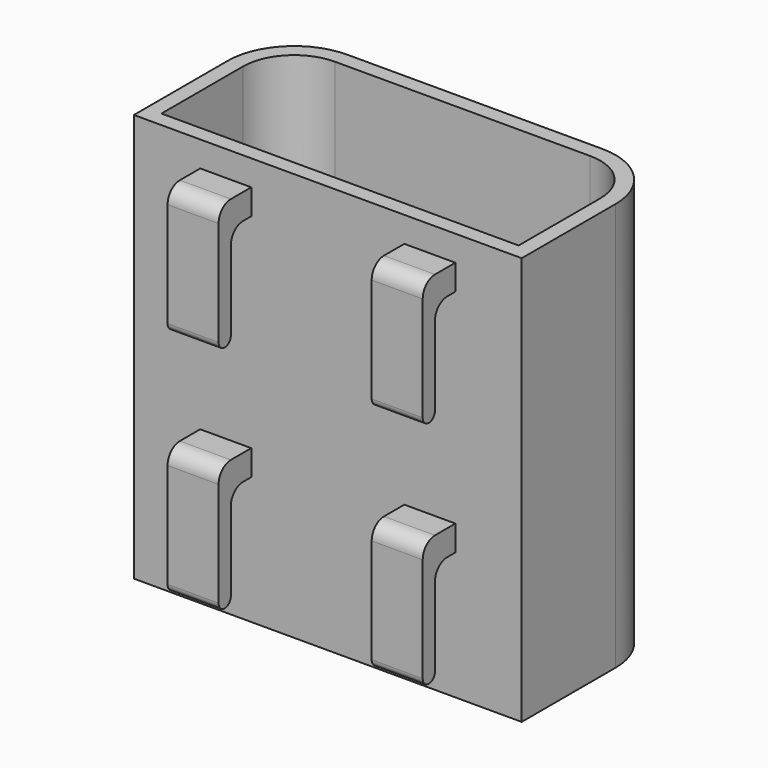
from build123d import *

# Parameters (mm, degrees)
F1_DEPTH = 80
F2_DEPTH = 3
F3_R     = 2.5
F4_DEPTH = 3
F5_W     = 10
F5_H     = 5
F6_DEPTH = 5
F7_W     = 10
F7_H     = 25
F8_DEPTH = 3
F9_R     = 3
F10_R    = 1.49999


# Not quite as in the source:
# - a fillet or chamfer is up to 0.001 mm smaller than in the source, because OpenCascade refuses the exact size


with BuildPart() as f1:
    # F0 (on Top) → F1 (new body)
    with BuildSketch(Plane.XY):
        with BuildLine():
            Line((-38, 5), (-38, -18))
            Line((-38, -18), (38, -18))
            Line((38, -18), (38, 5))
            ThreePointArc((38, 5), (34.1923881554, 14.1923881554), (25, 18))
            Line((25, 18), (-25, 18))
            ThreePointArc((-25, 18), (-34.1923881554, 14.1923881554), (-38, 5))
        make_face()
        with BuildLine():
            Line((35, -15), (-35, -15))
            Line((-35, -15), (-35, 5))
            ThreePointArc((-35, 5), (-32.0710678119, 12.0710678119), (-25, 15))
            Line((-25, 15), (25, 15))
            ThreePointArc((25, 15), (32.0710678119, 12.0710678119), (35, 5))
            Line((35, 5), (35, -15))
        make_face(mode=Mode.SUBTRACT)
    extrude(amount=F1_DEPTH)

    # F0 (on Top) → F2 (join)
    with BuildSketch(Plane.XY):
        with BuildLine():
            Line((-35, 5), (-35, -15))
            Line((-35, -15), (35, -15))
            Line((35, -15), (35, 5))
            ThreePointArc((35, 5), (32.0710678119, 12.0710678119), (25, 15))
            Line((25, 15), (-25, 15))
            ThreePointArc((-25, 15), (-32.0710678119, 12.0710678119), (-35, 5))
        make_face()
    extrude(amount=F2_DEPTH)

    # F3 (on face) → F4 (cut)
    with BuildSketch(Plane.XY.offset(3)):
        with BuildLine():
            ThreePointArc((-30.2998951749, 13.4800419301), (-28.5001310143, 10.050537004), (-25.5, 12.5))
            ThreePointArc((-25.5, 12.5), (-25.9114746987, 13.8740677079), (-27.0104496527, 14.7958201389))
            ThreePointArc((-27.0104496527, 14.7958201389), (-28.7139067635, 14.2847669089), (-30.2998951749, 13.4800419301))
        make_face()
        with BuildLine():
            ThreePointArc((23.5, 12.5), (22.767766953, 14.267766953), (21, 15))
            ThreePointArc((21, 15), (19.232233047, 10.732233047), (23.5, 12.5))
        make_face()
        with BuildLine():
            ThreePointArc((16.5, 12.5), (15.767766953, 14.267766953), (14, 15))
            ThreePointArc((14, 15), (12.232233047, 10.732233047), (16.5, 12.5))
        make_face()
        with BuildLine():
            ThreePointArc((9.5, 12.5), (8.7677669588, 14.2677669471), (7.0000000165, 15))
            ThreePointArc((7.0000000165, 15), (5.2322330412, 10.7322330529), (9.5, 12.5))
        make_face()
        with BuildLine():
            ThreePointArc((2.5, 12.5), (1.7677669531, 14.2677669529), (3e-10, 15))
            ThreePointArc((3e-10, 15), (-1.7677669531, 10.7322330471), (2.5, 12.5))
        make_face()
        with BuildLine():
            ThreePointArc((-4.5, 12.5), (-5.2322330412, 14.2677669471), (-6.9999999835, 15))
            ThreePointArc((-6.9999999835, 15), (-8.7677669588, 10.7322330529), (-4.5, 12.5))
        make_face()
        with BuildLine():
            ThreePointArc((-11.5, 12.5), (-12.2322330423, 14.2677669482), (-13.9999999867, 15))
            ThreePointArc((-13.9999999867, 15), (-15.7677669577, 10.7322330518), (-11.5, 12.5))
        make_face()
        with BuildLine():
            ThreePointArc((-18.5, 12.5), (-19.232233047, 14.267766953), (-21, 15))
            ThreePointArc((-21, 15), (-22.767766953, 10.732233047), (-18.5, 12.5))
        make_face()
        with BuildLine():
            ThreePointArc((-32.5, 0.3621778265), (-33.232233047, 2.1299447795), (-35, 2.8621778265))
            Line((-35, 2.8621778265), (-35, -2.1378221735))
            ThreePointArc((-35, -2.1378221735), (-33.232233047, -1.4055891265), (-32.5, 0.3621778265))
        make_face()
        with BuildLine():
            ThreePointArc((-32.5, -11.775644347), (-33.232233047, -10.0078773941), (-35, -9.275644347))
            Line((-35, -9.275644347), (-35, -14.275644347))
            ThreePointArc((-35, -14.275644347), (-33.232233047, -13.5434113), (-32.5, -11.775644347))
        make_face()
        with BuildLine():
            ThreePointArc((35, -9.275644347), (32.5, -11.775644347), (35, -14.275644347))
            Line((35, -14.275644347), (35, -9.275644347))
        make_face()
        with BuildLine():
            ThreePointArc((30.2998951749, 13.4800419301), (28.7139067635, 14.2847669089), (27.0104496527, 14.7958201389))
            ThreePointArc((27.0104496527, 14.7958201389), (26.6259322921, 10.4114746987), (30.5, 12.5))
            ThreePointArc((30.5, 12.5), (30.449462996, 13.0001310143), (30.2998951749, 13.4800419301))
        make_face()
        with BuildLine():
            ThreePointArc((35, 2.8621778265), (32.5, 0.3621778265), (35, -2.1378221735))
            Line((35, -2.1378221735), (35, 2.8621778265))
        make_face()
        with Locations((10.5, 6.4378221735)):
            Circle(F3_R)
        with Locations((-24.5, 6.4378221735)):
            Circle(F3_R)
        with Locations((-3.5, 6.4378221735)):
            Circle(F3_R)
        with Locations((24.5, 6.4378221735)):
            Circle(F3_R)
        with Locations((-17.5, 6.4378221735)):
            Circle(F3_R)
        with Locations((17.5, 6.4378221735)):
            Circle(F3_R)
        with Locations((3.5, 6.4378221735)):
            Circle(F3_R)
        with Locations((-31.5, 6.4378221735)):
            Circle(F3_R)
        with Locations((31.5, 6.4378221735)):
            Circle(F3_R)
        with Locations((-10.5, 6.4378221735)):
            Circle(F3_R)
        with Locations((31.5, -5.7)):
            Circle(F3_R)
        with Locations((28, 0.3621778265)):
            Circle(F3_R)
        with Locations((-14, 0.3621778265)):
            Circle(F3_R)
        with Locations((-31.5, -5.7)):
            Circle(F3_R)
        with Locations((-7, 0.3621778265)):
            Circle(F3_R)
        with Locations((0, 0.3621778265)):
            Circle(F3_R)
        with Locations((10.5, -5.7)):
            Circle(F3_R)
        with Locations((-21, 0.3621778265)):
            Circle(F3_R)
        with Locations((-28, 0.3621778265)):
            Circle(F3_R)
        with Locations((-10.5, -5.7)):
            Circle(F3_R)
        with Locations((17.5, -5.7)):
            Circle(F3_R)
        with Locations((-24.5, -5.7)):
            Circle(F3_R)
        with Locations((7, 0.3621778265)):
            Circle(F3_R)
        with Locations((-3.5, -5.7)):
            Circle(F3_R)
        with Locations((24.5, -5.7)):
            Circle(F3_R)
        with Locations((14, 0.3621778265)):
            Circle(F3_R)
        with Locations((21, 0.3621778265)):
            Circle(F3_R)
        with Locations((3.5, -5.7)):
            Circle(F3_R)
        with Locations((-17.5, -5.7)):
            Circle(F3_R)
        with Locations((28, -11.775644347)):
            Circle(F3_R)
        with Locations((-14, -11.775644347)):
            Circle(F3_R)
        with Locations((-7, -11.775644347)):
            Circle(F3_R)
        with Locations((0, -11.775644347)):
            Circle(F3_R)
        with Locations((-21, -11.775644347)):
            Circle(F3_R)
        with Locations((-28, -11.775644347)):
            Circle(F3_R)
        with Locations((7, -11.775644347)):
            Circle(F3_R)
        with Locations((14, -11.775644347)):
            Circle(F3_R)
        with Locations((21, -11.775644347)):
            Circle(F3_R)
    extrude(amount=-F4_DEPTH, mode=Mode.SUBTRACT)

    # F5 (on face) → F6 (join)
    with BuildSketch(Plane.XZ.offset(18)):
        with Locations((-20, 72.5)):
            Rectangle(F5_W, F5_H)
        with Locations((20, 72.5)):
            Rectangle(F5_W, F5_H)
        with Locations((20, 27.5)):
            Rectangle(F5_W, F5_H)
        with Locations((-20, 27.5)):
            Rectangle(F5_W, F5_H)
    extrude(amount=F6_DEPTH)

    # F7 (on face) → F8 (join)
    with BuildSketch(Plane.XZ.offset(23)):
        with Locations((-20, 62.5)):
            Rectangle(F7_W, F7_H)
        with Locations((20, 62.5)):
            Rectangle(F7_W, F7_H)
        with Locations((20, 17.5)):
            Rectangle(F7_W, F7_H)
        with Locations((-20, 17.5)):
            Rectangle(F7_W, F7_H)
    extrude(amount=F8_DEPTH)

    # F9
    f9_edges = [f1.edges().sort_by_distance(p)[0] for p in [
        (-20, -26, 30),
        (20, -26, 30),
        (-20, -26, 75),
        (20, -26, 75),
        (20, -23, 25),
        (20, -23, 70),
        (-20, -23, 70),
        (-20, -23, 25),
    ]]
    fillet(f9_edges, radius=F9_R)

    # F10 (radius 1.5 in the source; OpenCascade refuses exactly that, so slightly less here)
    f10_edges = [f1.edges().sort_by_distance(p)[0] for p in [
        (20, -26, 50),
        (20, -23, 50),
        (20, -23, 5),
        (-20, -26, 50),
        (-20, -23, 50),
        (-20, -23, 5),
        (-20, -26, 5),
        (20, -26, 5),
    ]]
    fillet(f10_edges, radius=F10_R)


solid = f1.part
